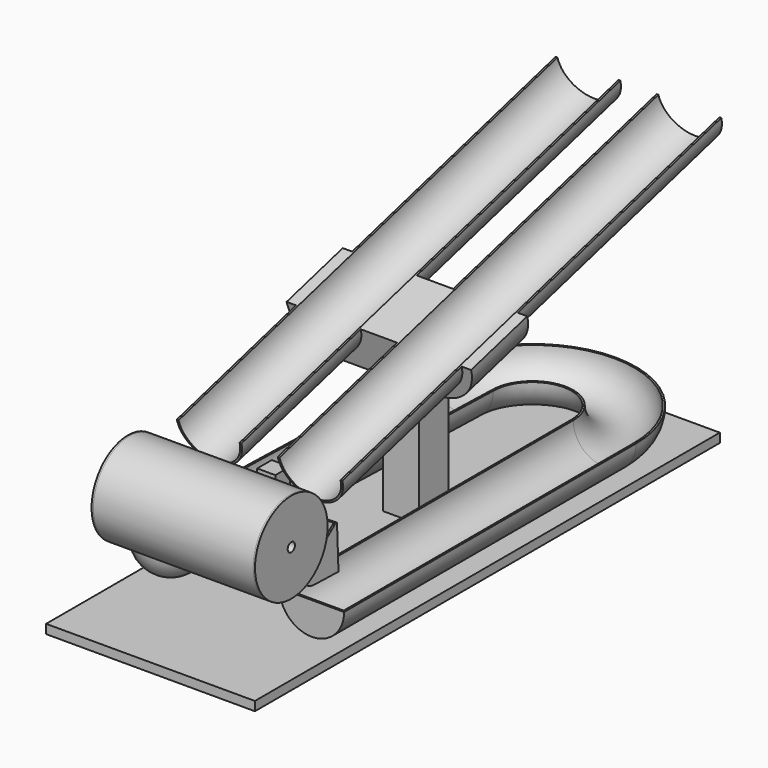
from build123d import *

# Parameters (mm, degrees)
F4_DEPTH  = 254
F8_DEPTH  = 1.27
F10_ANGLE = 180
F12_W     = 146.05
F12_H     = 406.4
F13_DEPTH = 6.35
F14_W     = 25.4
F14_H     = 25.4
F15_DEPTH = 101.6
F17_DEPTH = 85.726
F21_DEPTH = 25.4
F25_DEPTH = 171.45
F22_W     = 12.7
F22_H     = 12.7
F26_DEPTH = 76.2
F29_DEPTH = 41.275
F31_DEPTH = 1.27
F32_R     = 31.75
F33_DEPTH = 12.7
F35_DEPTH = 43.18
F37_DEPTH = 1.27
F38_R     = 3.175
F39_DEPTH = 130.176


# Not quite as in the source:
# - a pattern or mirror of a feature is missing from the dataset's text; its kind, count and spacing are read off the source's solid


with BuildPart() as f2:
    # F2: sweep along a path in F0
    with BuildLine(Plane.XY) as f2_path:
        ThreePointArc((49.911, 0), (0, 49.911), (-49.911, 0))
    # F1 (on Front) → F2 (sweep)
    with BuildSketch(Plane.XZ):
        with BuildLine():
            Line((-27.305, 0), (-28.575, 0))
            ThreePointArc((-28.575, 0), (-49.911, -21.336), (-71.247, 0))
            Line((-71.247, 0), (-72.517, 0))
            ThreePointArc((-72.517, 0), (-49.911, -22.606), (-27.305, 0))
        make_face()
    sweep(path=f2_path.line)

    # F4 (add): a face of the model
    f4_faces = [f2.faces().sort_by_distance(p)[0] for p in [
        (49.911, 0, -22.100514473),
    ]]
    extrude(f4_faces, amount=F4_DEPTH)

    # F6: sweep along a path in F5
    with BuildLine(Plane.YZ.offset(-49.911)) as f6_path:
        Line((0, 0), (-253.9206125938, 6.35))
    # F1 (on Front) → F6 (sweep)
    with BuildSketch(Plane.XZ):
        with BuildLine():
            Line((-27.305, 0), (-28.575, 0))
            ThreePointArc((-28.575, 0), (-49.911, -21.336), (-71.247, 0))
            Line((-71.247, 0), (-72.517, 0))
            ThreePointArc((-72.517, 0), (-49.911, -22.606), (-27.305, 0))
        make_face()
    sweep(path=f6_path.line)

    # F7 (on face) → F8 (join)
    with BuildSketch(Plane.XZ.offset(254)):
        with BuildLine():
            Line((28.575, 0), (27.305, 0))
            ThreePointArc((27.305, 0), (49.911, -22.606), (72.517, 0))
            Line((72.517, 0), (28.575, 0))
        make_face()
    extrude(amount=F8_DEPTH)

    # F9 (on face) → F10 (revolve)
    with BuildSketch(Plane.XZ.offset(253.9206125938)):
        with BuildLine():
            ThreePointArc((-49.911, -14.986), (-64.9978302834, -8.7368302834), (-71.247, 6.35))
            Line((-71.247, 6.35), (-72.517, 6.35))
            ThreePointArc((-72.517, 6.35), (-65.8958558955, -9.6348558955), (-49.911, -16.256))
            Line((-49.911, -16.256), (-49.911, -14.986))
        make_face()
    revolve(axis=Axis((-49.911, -253.9206125938, -14.6617003999), (0, 0, 1)), revolution_arc=F10_ANGLE)


with BuildPart() as f13:
    # F12 (on offset) → F13 (new body)
    with BuildSketch(Plane.XY.offset(-22.606)):
        with Locations((0, -130.683)):
            Rectangle(F12_W, F12_H)
    extrude(amount=-F13_DEPTH)

    # F14 (on face) → F15 (join)
    with BuildSketch(Plane.XY.offset(-22.606)):
        with Locations((0, -102.1575182676)):
            Rectangle(F14_W, F14_H)
    extrude(amount=F15_DEPTH)

    # F16 (on face) → F17 (cut, through all)
    with BuildSketch(Plane.YZ.offset(12.7)):
        Polygon((-114.8575182676, 72.1880905122), (-89.4575182676, 78.994), (-114.8575182676, 78.994), align=None)
    extrude(amount=-F17_DEPTH, mode=Mode.SUBTRACT)

    # F20 (on line) → F21 (join, symmetric)
    with BuildSketch(Plane(origin=(0, -76.4165008235, -20.4757396841), x_dir=(-1, 0, 0), z_dir=(0, 0.9659258263, 0.2588190451))):
        with BuildLine():
            Line((12.7, 128.6656541771), (-12.7, 128.6656541771))
            ThreePointArc((-12.7, 128.6656541771), (-35.306, 106.0596541771), (-57.912, 128.6656541771))
            Line((-57.912, 128.6656541771), (-64.516, 128.6656541771))
            ThreePointArc((-64.516, 128.6656541771), (-55.9605890785, 108.0110650987), (-35.306, 99.4556541771))
            Line((-35.306, 99.4556541771), (-12.7, 99.4556541771))
            Line((-12.7, 99.4556541771), (12.7, 99.4556541771))
            Line((12.7, 99.4556541771), (35.306, 99.4556541771))
            ThreePointArc((35.306, 99.4556541771), (55.9605890785, 108.0110650987), (64.516, 128.6656541771))
            Line((64.516, 128.6656541771), (57.912, 128.6656541771))
            ThreePointArc((57.912, 128.6656541771), (35.306, 106.0596541771), (12.7, 128.6656541771))
        make_face()
    extrude(amount=F21_DEPTH, both=True)

    # F24 (on offset) → F25 (join, symmetric)
    with BuildSketch(Plane(origin=(0, -39.6147268418, -10.6147340657), x_dir=(-1, 0, 0), z_dir=(0, 0.9659258263, 0.2588190451))):
        with BuildLine():
            ThreePointArc((12.7, 128.6656541771), (35.306, 106.0596541771), (57.912, 128.6656541771))
            Line((57.912, 128.6656541771), (56.642, 128.6656541771))
            ThreePointArc((56.642, 128.6656541771), (35.306, 107.3296541771), (13.97, 128.6656541771))
            Line((13.97, 128.6656541771), (12.7, 128.6656541771))
        make_face()
        with BuildLine():
            ThreePointArc((-57.912, 128.6656541771), (-35.306, 106.0596541771), (-12.7, 128.6656541771))
            Line((-12.7, 128.6656541771), (-13.97, 128.6656541771))
            ThreePointArc((-13.97, 128.6656541771), (-35.306, 107.3296541771), (-56.642, 128.6656541771))
            Line((-56.642, 128.6656541771), (-57.912, 128.6656541771))
        make_face()
    extrude(amount=F25_DEPTH, both=True)

    # F22 (on offset) → F26 (join)
    with BuildSketch(Plane.XY.offset(-22.606)):
        with Locations((0, -226.314)):
            Rectangle(F22_W, F22_H)
    extrude(amount=F26_DEPTH)


with BuildPart() as f29:
    # F28 (on face) → F29 (new body, symmetric)
    with BuildSketch(Plane(origin=(8.2115300865, 0, 0.2867529493), x_dir=(0, 1, 0), z_dir=(0.999390827, 0, 0.0348994967))):
        with BuildLine():
            Line((-253.9206125938, 7.299062509), (-232.664, 6.7678048741))
            Line((-232.664, 6.7678048741), (-232.664, 36.6892963648))
            Line((-232.664, 36.6892963648), (-233.934, 36.6892963648))
            Line((-233.934, 36.6892963648), (-233.934, 8.0699420309))
            Line((-233.934, 8.0699420309), (-253.8888819229, 8.5686660552))
            ThreePointArc((-253.8888819229, 8.5686660552), (-259.4287437221, 10.365927761), (-263.0892697017, 14.8959131855))
            Line((-263.0892697017, 14.8959131855), (-264.2679131519, 14.4228155679))
            ThreePointArc((-264.2679131519, 14.4228155679), (-260.1532069871, 9.322815393), (-253.9206125938, 7.299062509))
        make_face()
    extrude(amount=F29_DEPTH, both=True)

    # F30 (on face) → F31 (join)
    with BuildSketch(Plane(origin=(49.4613864717, 0, 1.7272296757), x_dir=(0, 1, 0), z_dir=(0.999390827, 0, 0.0348994967))):
        with BuildLine():
            Line((-232.664, 36.6892963648), (-233.934, 36.6892963648))
            Line((-233.934, 36.6892963648), (-233.934, 8.0699420309))
            Line((-233.934, 8.0699420309), (-253.8888819229, 8.5686660552))
            ThreePointArc((-253.8888819229, 8.5686660552), (-259.4287437221, 10.365927761), (-263.0892697017, 14.8959131855))
            Line((-263.0892697017, 14.8959131855), (-264.2679131519, 14.4228155679))
            ThreePointArc((-264.2679131519, 14.4228155679), (-260.1532069871, 9.322815393), (-253.9206125938, 7.299062509))
            Line((-253.9206125938, 7.299062509), (-232.664, 6.7678048741))
            Line((-232.664, 6.7678048741), (-232.664, 36.6892963648))
        make_face()
        with BuildLine():
            Line((-233.934, 8.0699420309), (-233.934, 36.6892963648))
            Line((-233.934, 36.6892963648), (-263.0892697017, 14.8959131855))
            ThreePointArc((-263.0892697017, 14.8959131855), (-259.4287437221, 10.365927761), (-253.8888819229, 8.5686660552))
            Line((-253.8888819229, 8.5686660552), (-233.934, 8.0699420309))
        make_face()
    extrude(amount=F31_DEPTH)


with BuildPart() as f33:
    # F32 (on Right) → F33 (new body, symmetric)
    with BuildSketch(Plane.YZ):
        with Locations((-282.2139802206, 45.8837522464)):
            Circle(F32_R)
    extrude(amount=F33_DEPTH, both=True)

    # F34 (on face) → F35 (join)
    with BuildSketch(Plane.YZ.offset(12.7)):
        with BuildLine():
            Line((-271.6438700154, 57.9873626296), (-263.8157591623, 71.7597635675))
            ThreePointArc((-263.8157591623, 71.7597635675), (-310.851300877, 32.17366962), (-250.5205643565, 43.9890515145))
            ThreePointArc((-250.5205643565, 43.9890515145), (-267.6183225651, 41.1252921384), (-271.6438700154, 57.9873626296))
        make_face()
    f35 = extrude(amount=F35_DEPTH)

    # F35_copies: F35 across plane
    add(f35.mirror(Plane(origin=(0, 0, 0), x_dir=(0, 0, -1), z_dir=(-1, 0, 0))))

    # F36 (on face) → F37 (join)
    with BuildSketch(Plane.YZ.offset(55.88)):
        with BuildLine():
            ThreePointArc((-250.5205643565, 43.9890515145), (-253.5766595643, 59.5938348729), (-263.8157591623, 71.7597635675))
            Line((-263.8157591623, 71.7597635675), (-271.6438700154, 57.9873626296))
            ThreePointArc((-271.6438700154, 57.9873626296), (-267.6183225651, 41.1252921384), (-250.5205643565, 43.9890515145))
        make_face()
        with BuildLine():
            Line((-271.6438700154, 57.9873626296), (-263.8157591623, 71.7597635675))
            ThreePointArc((-263.8157591623, 71.7597635675), (-310.851300877, 32.17366962), (-250.5205643565, 43.9890515145))
            ThreePointArc((-250.5205643565, 43.9890515145), (-267.6183225651, 41.1252921384), (-271.6438700154, 57.9873626296))
        make_face()
    f37 = extrude(amount=F37_DEPTH)

    # F37_copies: F37 across plane
    add(f37.mirror(Plane(origin=(0, 0, 0), x_dir=(0, 0, -1), z_dir=(-1, 0, 0))))

    # F38 (on face) → F39 (cut, through all)
    with BuildSketch(Plane.YZ.offset(57.15)):
        with Locations((-282.2139802206, 45.8837522464)):
            Circle(F38_R)
    extrude(amount=-F39_DEPTH, mode=Mode.SUBTRACT)


solid = Compound([f2.part, f13.part, f29.part, f33.part])
